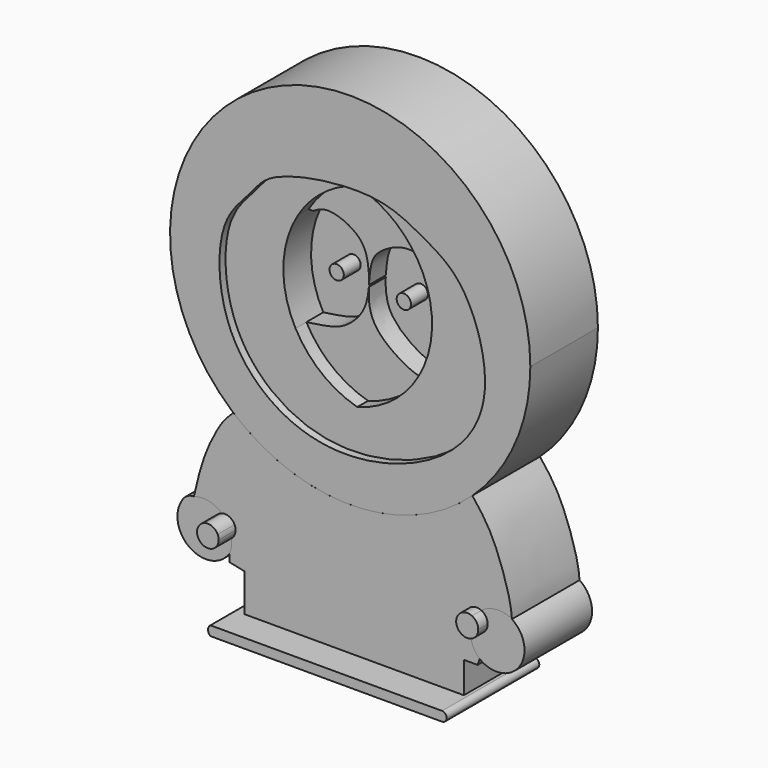
from build123d import *

# Parameters (mm, degrees)
F1_DEPTH = 25.4
F2_DEPTH = 19.05
F0_R     = 2.1462525612
F0_R_2   = 2.1514214695
F3_DEPTH = 12.7
F4_DEPTH = 23.114
F5_DEPTH = 28.956
F6_DEPTH = 34.798
F7_DEPTH = 25.4
F8_DEPTH = 31.75


with BuildPart() as f1:
    # F0 (on Front) → F1 (new body)
    with BuildSketch(Plane.XZ):
        with BuildLine():
            ThreePointArc((-38.8648257064, -47.8244096014), (-42.8447911552, -45.8517880459), (-47.2795665264, -46.1050234735))
            ThreePointArc((-47.2795665264, -46.1050234735), (-49.4417962283, -46.7561522698), (-50.9271398187, -48.4570227563))
            ThreePointArc((-50.9271398187, -48.4570227563), (-48.3270967212, -60.184982173), (-36.5713872015, -57.7134341002))
            ThreePointArc((-36.5713872015, -57.7134341002), (-35.9927494085, -55.6381951602), (-35.9427130647, -53.484376524))
            ThreePointArc((-35.9427130647, -53.484376524), (-40.8914655293, -52.4550115347), (-38.8648257064, -47.8244096014))
        make_face()
    extrude(amount=F1_DEPTH)


with BuildPart() as f1b:
    # F0 (on Front) → F1, piece 2 (new body)
    with BuildSketch(Plane.XZ):
        with BuildLine():
            ThreePointArc((38.6058650911, -61.149969697), (50.5575613316, -59.3662033207), (48.3456142247, -47.4862977862))
            ThreePointArc((48.3456142247, -47.4862977862), (43.6507360707, -46.4589475822), (39.1555038082, -48.1590111775))
            ThreePointArc((39.1555038082, -48.1590111775), (40.5422324312, -49.3834370221), (41.0578993444, -51.1600412428))
            ThreePointArc((41.0578993444, -51.1600412428), (39.2941563686, -54.0916500414), (35.8778789209, -53.9068046115))
            ThreePointArc((35.8778789209, -53.9068046115), (36.3633487173, -57.8592645198), (38.6058650911, -61.149969697))
        make_face()
    extrude(amount=F1_DEPTH)

    # F0 (on Front) → F5 (join)
    with BuildSketch(Plane.XZ):
        with BuildLine():
            ThreePointArc((41.0578993444, -51.1600412428), (40.5422324312, -49.3834370221), (39.1555038082, -48.1590111775))
            ThreePointArc((39.1555038082, -48.1590111775), (34.8571067738, -49.5163049155), (35.8778789209, -53.9068046115))
            ThreePointArc((35.8778789209, -53.9068046115), (39.2941563686, -54.0916500414), (41.0578993444, -51.1600412428))
        make_face()
    extrude(amount=F5_DEPTH)


with BuildPart() as f1c:
    # F0 (on Front) → F1, piece 3 (new body)
    with BuildSketch(Plane.XZ):
        with BuildLine():
            ThreePointArc((36.4421369612, -18.6651921315), (49.3201130573, -0.5904283353), (53.8672931298, 21.1319681257))
            ThreePointArc((53.8672931298, 21.1319681257), (-22.9913845707, 70.3039772139), (-35.4215330811, -20.0875833636))
            ThreePointArc((-35.4215330811, -20.0875833636), (0.7802734495, -33.0161958648), (36.4421369612, -18.6651921315))
        make_face()
        with BuildLine():
            add(Edge.make_bspline(
                [(-30.4386503994, 39.5811572671), (-32.774598956, 36.8594468694), (-40.6208067301, 29.8814035553), (-39.9167404184, 1.4186076865), (-21.8901689435, -17.7941397611), (3.4211558325, -22.2897317842), (31.0854974178, -11.8183159889), (43.9988092966, 9.6949162526), (34.8024966241, 37.6219194181), (21.349404744, 44.9621968255), (7.2103582856, 53.1156372047), (-24.6572111467, 48.1787281069), (-28.4063082123, 41.9491233112), (-30.4386503994, 39.5811572671)],
                knots=[0, 0, 0, 0, 0.0710411926, 0.1726859002, 0.2717459946, 0.3700612246, 0.4754764407, 0.5707842376, 0.673296182, 0.7486675962, 0.8292657243, 0.9381921265, 1, 1, 1, 1], degree=3))
        make_face(mode=Mode.SUBTRACT)
    extrude(amount=F1_DEPTH)


with BuildPart() as f2:
    # F0 (on Front) → F2 (new body)
    with BuildSketch(Plane.XZ):
        with BuildLine():
            add(Edge.make_bspline(
                [(19.7713409874, 33.8124296001), (17.0530017987, 35.0664739659), (11.5213178042, 37.6093098644), (2.333806827, 32.4805735345), (0.7752005326, 28.2282579362), (0.403500899, 24.9385996088), (0.2726573334, 22.7563486921)],
                knots=[0, 0, 0, 0, 0.1541827795, 0.3132276804, 0.419976068, 0.542256765, 0.542256765, 0.542256765, 0.542256765], degree=3))
            ThreePointArc((19.7713409874, 33.8124296001), (11.7607731404, 44.3834894386), (0, 50.5154319108))
            ThreePointArc((0, 50.5154319108), (-10.2469715932, 45.4194091459), (-17.8808216998, 36.8933193386))
            Line((-17.8808216998, 36.8933193386), (-16.5719501674, 36.8933193386))
            add(Edge.make_bspline(
                [(-16.5719501674, 36.8933193386), (-15.2309208835, 37.6677308186), (-12.0167478432, 39.5238339537), (-2.1170965477, 35.4435792475), (0.0300794173, 29.6572488333), (0.3551548845, 24.5978568848), (0.2726573336, 22.7563487051)],
                knots=[0, 0, 0, 0, 0.1140099411, 0.2731404719, 0.4152523762, 0.4954652578, 0.4954652578, 0.4954652578, 0.4954652578], degree=3))
        make_face()
    extrude(amount=F2_DEPTH)


with BuildPart() as f2b:
    # F0 (on Front) → F2, piece 2 (new body)
    with BuildSketch(Plane.XZ):
        with BuildLine():
            ThreePointArc((-18.5498786492, 6.7970533631), (-10.7793949698, -2.4866325596), (0, -7.9977018759))
            ThreePointArc((0, -7.9977018759), (9.3386246625, -3.7114990643), (16.7055176482, 3.4516240579))
            add(Edge.make_bspline(
                [(0.2421217657, 22.2079030234), (0.0955639093, 19.3182224693), (0.2689025379, 11.4097076559), (13.0914353168, 3.7243688962), (15.8143117845, 3.5152306101), (16.7055176482, 3.4516240579)],
                knots=[0.5523432893, 0.5523432893, 0.5523432893, 0.5523432893, 0.7094395409, 0.9045152153, 1, 1, 1, 1], degree=3))
            add(Edge.make_bspline(
                [(0.2421217657, 22.2079030234), (0.1056898884, 20.1627042788), (-0.9553729768, 14.6433520503), (-6.4653297888, 9.54568452), (-11.2512681006, 7.8548837498), (-15.9699969863, 7.166375328), (-18.5498786492, 6.7970533631)],
                knots=[0.5034243416, 0.5034243416, 0.5034243416, 0.5034243416, 0.5924517916, 0.744271431, 0.8596311559, 1, 1, 1, 1], degree=3))
        make_face()
    extrude(amount=F2_DEPTH)


with BuildPart() as f2c:
    # F0 (on Front) → F2, piece 3 (new body)
    with BuildSketch(Plane.XZ):
        with Locations((-9.4405384734, 22.9637362063)):
            Circle(F0_R)
    extrude(amount=F2_DEPTH)


with BuildPart() as f2d:
    # F0 (on Front) → F2, piece 4 (new body)
    with BuildSketch(Plane.XZ):
        with Locations((10.754021816, 21.7640604824)):
            Circle(F0_R_2)
    extrude(amount=F2_DEPTH)


with BuildPart() as f3:
    # F0 (on Front) → F3 (new body)
    with BuildSketch(Plane.XZ):
        with BuildLine():
            ThreePointArc((-17.8808216998, 36.8933193386), (-22.2062923095, 21.9339072431), (-18.5498786492, 6.7970533631))
            add(Edge.make_bspline(
                [(0.2421217657, 22.2079030234), (0.1056898884, 20.1627042788), (-0.9553729768, 14.6433520503), (-6.4653297888, 9.54568452), (-11.2512681006, 7.8548837498), (-15.9699969863, 7.166375328), (-18.5498786492, 6.7970533631)],
                knots=[0.5034243416, 0.5034243416, 0.5034243416, 0.5034243416, 0.5924517916, 0.744271431, 0.8596311559, 1, 1, 1, 1], degree=3))
            add(Edge.make_bspline(
                [(0.2726573334, 22.7563486921), (0.2618644866, 22.5763421356), (0.251531663, 22.393437922), (0.242121767, 22.2079030476)],
                knots=[0.542256765, 0.542256765, 0.542256765, 0.542256765, 0.5523432893, 0.5523432893, 0.5523432893, 0.5523432893], degree=3))
            add(Edge.make_bspline(
                [(-16.5719501674, 36.8933193386), (-15.2309208835, 37.6677308186), (-12.0167478432, 39.5238339537), (-2.1170965477, 35.4435792475), (0.0300794173, 29.6572488333), (0.3551548845, 24.5978568848), (0.2726573336, 22.7563487051)],
                knots=[0, 0, 0, 0, 0.1140099411, 0.2731404719, 0.4152523762, 0.4954652578, 0.4954652578, 0.4954652578, 0.4954652578], degree=3))
            Line((-16.5719501674, 36.8933193386), (-17.8808216998, 36.8933193386))
        make_face()
        with Locations((-9.4405384734, 22.9637362063)):
            Circle(F0_R, mode=Mode.SUBTRACT)
    extrude(amount=F3_DEPTH)


with BuildPart() as f3b:
    # F0 (on Front) → F3, piece 2 (new body)
    with BuildSketch(Plane.XZ):
        with BuildLine():
            add(Edge.make_bspline(
                [(0.2421217657, 22.2079030234), (0.0955639093, 19.3182224693), (0.2689025379, 11.4097076559), (13.0914353168, 3.7243688962), (15.8143117845, 3.5152306101), (16.7055176482, 3.4516240579)],
                knots=[0.5523432893, 0.5523432893, 0.5523432893, 0.5523432893, 0.7094395409, 0.9045152153, 1, 1, 1, 1], degree=3))
            ThreePointArc((16.7055176482, 3.4516240579), (22.3438016033, 18.2174677966), (19.7713409874, 33.8124296001))
            add(Edge.make_bspline(
                [(19.7713409874, 33.8124296001), (17.0530017987, 35.0664739659), (11.5213178042, 37.6093098644), (2.333806827, 32.4805735345), (0.7752005326, 28.2282579362), (0.403500899, 24.9385996088), (0.2726573334, 22.7563486921)],
                knots=[0, 0, 0, 0, 0.1541827795, 0.3132276804, 0.419976068, 0.542256765, 0.542256765, 0.542256765, 0.542256765], degree=3))
            add(Edge.make_bspline(
                [(0.2726573336, 22.7563487051), (0.2644715545, 22.5736259591), (0.2543188212, 22.3907444758), (0.2421217657, 22.2079030234)],
                knots=[0.4954652578, 0.4954652578, 0.4954652578, 0.4954652578, 0.5034243416, 0.5034243416, 0.5034243416, 0.5034243416], degree=3))
        make_face()
        with Locations((10.754021816, 21.7640604824)):
            Circle(F0_R_2, mode=Mode.SUBTRACT)
    extrude(amount=F3_DEPTH)


with BuildPart() as f4:
    # F0 (on Front) → F4 (new body)
    with BuildSketch(Plane.XZ):
        with BuildLine():
            add(Edge.make_bspline(
                [(-30.4386503994, 39.5811572671), (-32.774598956, 36.8594468694), (-40.6208067301, 29.8814035553), (-39.9167404184, 1.4186076865), (-21.8901689435, -17.7941397611), (3.4211558325, -22.2897317842), (31.0854974178, -11.8183159889), (43.9988092966, 9.6949162526), (34.8024966241, 37.6219194181), (21.349404744, 44.9621968255), (7.2103582856, 53.1156372047), (-24.6572111467, 48.1787281069), (-28.4063082123, 41.9491233112), (-30.4386503994, 39.5811572671)],
                knots=[0, 0, 0, 0, 0.0710411926, 0.1726859002, 0.2717459946, 0.3700612246, 0.4754764407, 0.5707842376, 0.673296182, 0.7486675962, 0.8292657243, 0.9381921265, 1, 1, 1, 1], degree=3))
        make_face()
        with BuildLine():
            ThreePointArc((16.7055176482, 3.4516240579), (9.3386246625, -3.7114990643), (0, -7.9977018759))
            ThreePointArc((0, -7.9977018759), (-10.7793949698, -2.4866325596), (-18.5498786492, 6.7970533631))
            ThreePointArc((-18.5498786492, 6.7970533631), (-22.2062923095, 21.9339072431), (-17.8808216998, 36.8933193386))
            ThreePointArc((-17.8808216998, 36.8933193386), (-10.2469715932, 45.4194091459), (0, 50.5154319108))
            ThreePointArc((0, 50.5154319108), (11.7607731404, 44.3834894386), (19.7713409874, 33.8124296001))
            ThreePointArc((19.7713409874, 33.8124296001), (22.3438016033, 18.2174677966), (16.7055176482, 3.4516240579))
        make_face(mode=Mode.SUBTRACT)
    extrude(amount=F4_DEPTH)


with BuildPart() as f6:
    # F0 (on Front) → F6 (new body)
    with BuildSketch(Plane.XZ):
        with BuildLine():
            Line((34.8290167749, -72.3302215338), (33.878352493, -72.3302215338))
            Line((33.878352493, -72.3302215338), (-32.0263206959, -72.3302215338))
            Line((-32.0263206959, -72.3302215338), (-34.7852036357, -72.3302215338))
            ThreePointArc((-34.7852036357, -72.3302215338), (-35.512709611, -73.7636759877), (-34.7852036357, -75.1971304417))
            Line((-34.7852036357, -75.1971304417), (34.8100066185, -75.1971304417))
            ThreePointArc((34.8100066185, -75.1971304417), (36.2434925857, -73.7731182478), (34.8290167749, -72.3302215338))
        make_face()
    extrude(amount=F6_DEPTH)


with BuildPart() as f7:
    # F0 (on Front) → F7 (new body)
    with BuildSketch(Plane.XZ):
        with BuildLine():
            ThreePointArc((36.4421369612, -18.6651921315), (0.7802734495, -33.0161958648), (-35.4215330811, -20.0875833636))
            add(Edge.make_bspline(
                [(-47.2795665264, -46.1050234735), (-46.3125634164, -41.8947026932), (-44.4864239912, -33.9453719385), (-39.4951734191, -24.4891424364), (-37.3499339141, -22.0530112025), (-36.0489577996, -20.7277891737), (-35.4215330811, -20.0875833636)],
                knots=[0, 0, 0, 0, 0.3534329239, 0.6678249179, 0.8408647615, 1, 1, 1, 1], degree=3))
            ThreePointArc((-47.2795665264, -46.1050234735), (-42.8447911552, -45.8517880459), (-38.8648257064, -47.8244096014))
            ThreePointArc((-38.8648257064, -47.8244096014), (-36.6303494384, -48.0092356193), (-35.0456094113, -49.5953137685))
            ThreePointArc((-35.0456094113, -49.5953137685), (-34.8208828003, -50.2622673454), (-34.7447878545, -50.9619377553))
            ThreePointArc((-34.7447878545, -50.9619377553), (-35.0594831205, -52.3581578446), (-35.9427130647, -53.484376524))
            ThreePointArc((-35.9427130647, -53.484376524), (-35.9927494085, -55.6381951602), (-36.5713872015, -57.7134341002))
            Line((-36.5713872015, -57.7134341002), (-36.5713872015, -60.0413940847))
            Line((-36.5713872015, -60.0413940847), (-32.0263206959, -60.9836652875))
            Line((-32.0263206959, -60.9836652875), (-32.0263206959, -72.3302215338))
            Line((-32.0263206959, -72.3302215338), (33.878352493, -72.3302215338))
            Line((33.878352493, -72.3302215338), (33.878352493, -62.9545077682))
            Line((33.878352493, -62.9545077682), (38.0453057587, -62.9545077682))
            Line((38.0453057587, -62.9545077682), (38.6058650911, -61.149969697))
            ThreePointArc((38.6058650911, -61.149969697), (36.3633487173, -57.8592645198), (35.8778789209, -53.9068046115))
            ThreePointArc((35.8778789209, -53.9068046115), (34.8571067738, -49.5163049155), (39.1555038082, -48.1590111775))
            ThreePointArc((39.1555038082, -48.1590111775), (43.6507360707, -46.4589475822), (48.3456142247, -47.4862977862))
            add(Edge.make_bspline(
                [(36.4421369612, -18.6651921315), (38.4667538868, -21.2271465393), (42.921184752, -26.8809508094), (47.9228736043, -42.280547663), (48.2332466792, -46.1090309228), (48.3456142247, -47.4862977862)],
                knots=[0, 0, 0, 0, 0.3445026937, 0.7646391486, 1, 1, 1, 1], degree=3))
        make_face()
    extrude(amount=F7_DEPTH)


with BuildPart() as f8:
    # F0 (on Front) → F8 (new body)
    with BuildSketch(Plane.XZ):
        with BuildLine():
            ThreePointArc((-35.0456094113, -49.5953137685), (-36.6303494384, -48.0092356193), (-38.8648257064, -47.8244096014))
            ThreePointArc((-38.8648257064, -47.8244096014), (-40.8914655293, -52.4550115347), (-35.9427130647, -53.484376524))
            ThreePointArc((-35.9427130647, -53.484376524), (-35.0594831205, -52.3581578446), (-34.7447878545, -50.9619377553))
            ThreePointArc((-34.7447878545, -50.9619377553), (-34.8208828003, -50.2622673454), (-35.0456094113, -49.5953137685))
        make_face()
    extrude(amount=F8_DEPTH)


solid = Compound([f1.part, f1b.part, f1c.part, f2.part, f2b.part, f2c.part, f2d.part, f3.part, f3b.part, f4.part, f6.part, f7.part, f8.part])
